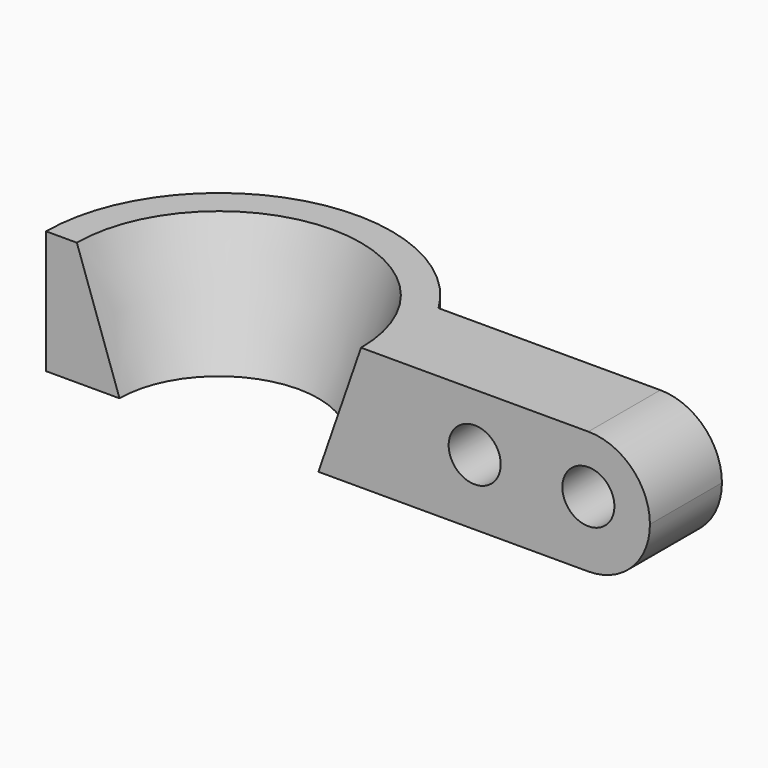
from build123d import *

# Parameters (mm, degrees)
F1_DEPTH = 52
F4_R     = 11
F5_DEPTH = 154
F6_R     = 25.99999


# Not quite as in the source:
# - a fillet or chamfer is up to 0.001 mm smaller than in the source, because OpenCascade refuses the exact size


with BuildPart() as f1:
    # F0 (on Top) → F1 (new body)
    with BuildSketch(Plane.XY):
        with BuildLine():
            ThreePointArc((-42, 0), (0, 42), (42, 0))
            Line((42, 0), (73, 0))
            Line((73, 0), (182, 0))
            Line((182, 0), (182, 38))
            Line((182, 38), (62.329768169, 38))
            ThreePointArc((62.329768169, 38), (-19.7348286497, 70.2818364741), (-73, 0))
            Line((-73, 0), (-42, 0))
        make_face()
    extrude(amount=F1_DEPTH)

    # F2 (on face) → F3 (revolve, cut)
    with BuildSketch(Plane.XZ):
        Polygon((-42, 52), (-60, 52), (-42, 0), align=None)
    revolve(axis=Axis((0, 0, 25.9652175009), (0, 0, -1)), mode=Mode.SUBTRACT)

    # F4 (on face) → F5 (cut)
    with BuildSketch(Plane.XZ):
        with Locations((108, 27.769446373)):
            Circle(F4_R)
        with Locations((156, 27.8078082746)):
            Circle(F4_R)
    extrude(amount=-F5_DEPTH, mode=Mode.SUBTRACT)

    # F6 (radius 26 in the source; OpenCascade refuses exactly that, so slightly less here)
    f6_edges = [f1.edges().sort_by_distance(p)[0] for p in [
        (182, 19, 52),
        (182, 19, 0),
    ]]
    fillet(f6_edges, radius=F6_R)


solid = f1.part
